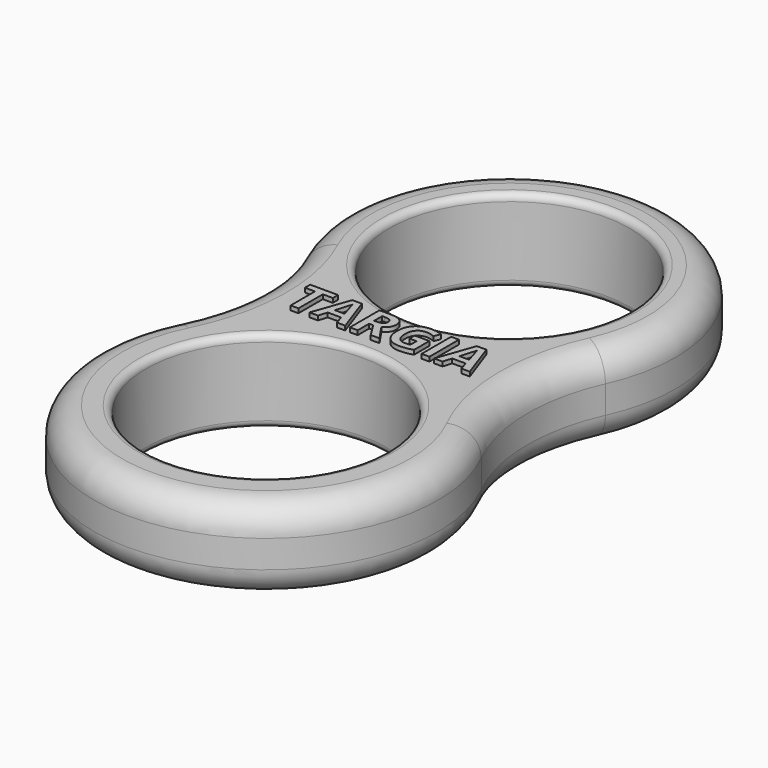
from build123d import *

# Parameters (mm, degrees)
F0_R         = 11.049
F1_DEPTH     = 7.62
F2_R         = 2.54
F3_R         = 0.635
F4_TEXT_SIZE = 4.7550039697
F5_DEPTH     = 0.396875


# Not quite as in the source:
# - Text() gives the source's letters only with a copy of the font that has no kerning and outlines rounded to 1/6400 em; it was checked with that copy


with BuildPart() as f1:
    # F0 (on Top) → F1 (new body)
    with BuildSketch(Plane.XY):
        with BuildLine():
            ThreePointArc((14.1259655302, 7.0487873604), (12.3480350241, 14.3059890852), (13.868448415, 21.6214765521))
            ThreePointArc((13.868448415, 21.6214765521), (0, 43.18), (-13.868448415, 21.6214765521))
            ThreePointArc((-13.868448415, 21.6214765521), (-12.3480350241, 14.3059890852), (-14.1259655302, 7.0487873604))
            ThreePointArc((-14.1259655302, 7.0487873604), (0, -15.7869663145), (14.1259655302, 7.0487873604))
        make_face()
        Circle(F0_R, mode=Mode.SUBTRACT)
        with Locations((0, 27.94)):
            Circle(F0_R, mode=Mode.SUBTRACT)
    extrude(amount=F1_DEPTH)

    # F2
    f2_edges = [f1.edges().sort_by_distance(p)[0] for p in [
        (12.348035, 14.305989, 7.62),
        (12.348035, 14.305989, 0),
    ]]
    fillet(f2_edges, radius=F2_R)

    # F3
    f3_edges = [f1.edges().sort_by_distance(p)[0] for p in [
        (-11.049, 0, 7.62),
        (-11.049, 27.94, 7.62),
        (-11.049, 0, 0),
        (-11.049, 27.94, 0),
    ]]
    fillet(f3_edges, radius=F3_R)

    # F4 (on face) → F5 (join)
    with BuildSketch(Plane.XY.offset(7.62)):
        with Locations((-8.8598581491, 12.6248285812)):
            Text('TARGIA', F4_TEXT_SIZE, font='Open Sans', font_style=FontStyle.BOLD, text_align=(TextAlign.LEFT, TextAlign.BOTTOM))
    extrude(amount=F5_DEPTH)


solid = f1.part
